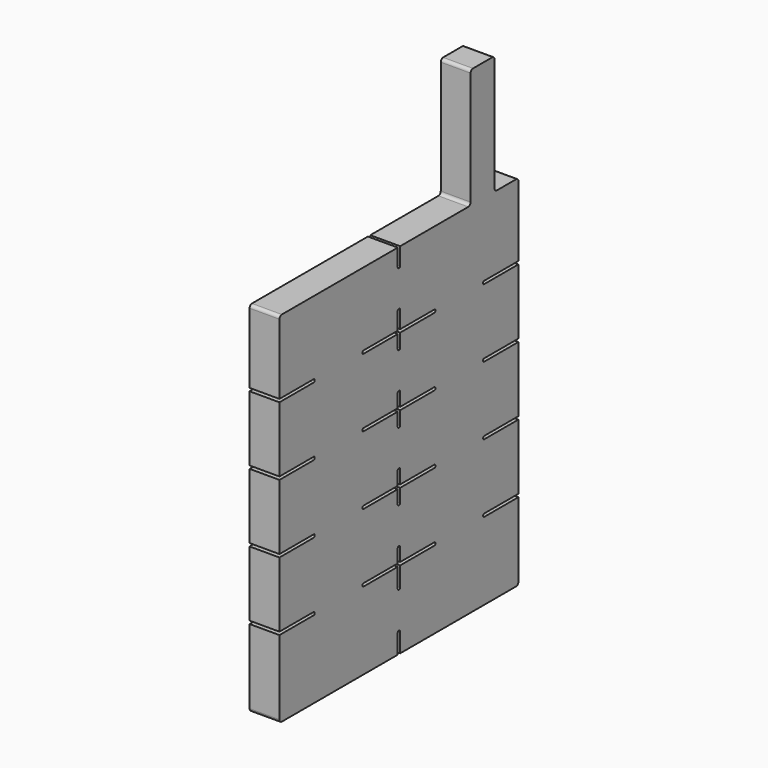
from build123d import *

# Parameters (mm, degrees)
F1_DEPTH = 5
F2_R     = 0.5
F3_R     = 0.5
F4_R     = 0.5
F5_R     = 0.2


# Not quite as in the source:
# - a feature names something its author has since deleted; it is built from what else it names


with BuildPart() as f1:
    # F0 (on Right) → F1 (new body)
    with BuildSketch(Plane.YZ):
        Polygon((11.5, 0), (0, 0), (0, -12.238), (7.3750000447, -12.238), (7.3750000447, -12.738), (0, -12.738), (0, -23.672), (7.3750000447, -23.672), (7.3750000447, -24.172), (0, -24.172), (0, -35.106), (7.3750000447, -35.106), (7.3750000447, -35.606), (0, -35.606), (0, -46.54), (7.3750000447, -46.54), (7.3750000447, -47.04), (0, -47.04), (0, -60), (24.75, -60), (24.75, -56.52), (25.25, -56.52), (25.25, -60), (50, -60), (50, -47.04), (42.6249988377, -47.04), (42.6249988377, -46.54), (50, -46.54), (50, -35.606), (42.6249988377, -35.606), (42.6249988377, -35.106), (50, -35.106), (50, -24.172), (42.6249988377, -24.172), (42.6249988377, -23.672), (50, -23.672), (50, -12.738), (42.6249988377, -12.738), (42.6249988377, -12.238), (50, -12.238), (50, 0), (45, 0), (45, 15), (45, 19.999999553), (40, 19.999999553), (40, 15), (40, 0), (37.625, 0), (35.125, 0), (25.25, 0), (25.25, -1.304), (25.25, -3.119), (24.75, -3.119), (24.75, 0), (14.875, 0), (12.375, 0), align=None)
        Polygon((25.25, -44.073), (25.25, -46.54), (32.625, -46.54), (32.625, -47.04), (25.25, -47.04), (25.25, -50.52), (24.75, -50.52), (24.75, -47.04), (17.375, -47.04), (17.375, -46.54), (24.75, -46.54), (24.75, -44.073), align=None, mode=Mode.SUBTRACT)
        Polygon((25.25, -32.639), (25.25, -35.106), (32.625, -35.106), (32.625, -35.606), (25.25, -35.606), (25.25, -38.073), (24.75, -38.073), (24.75, -35.606), (17.375, -35.606), (17.375, -35.106), (24.75, -35.106), (24.75, -32.639), align=None, mode=Mode.SUBTRACT)
        Polygon((25.25, -21.205), (25.25, -23.672), (32.625, -23.672), (32.625, -24.172), (25.25, -24.172), (25.25, -26.639), (24.75, -26.639), (24.75, -24.172), (17.375, -24.172), (17.375, -23.672), (24.75, -23.672), (24.75, -21.205), align=None, mode=Mode.SUBTRACT)
        Polygon((25.25, -9.119), (25.25, -12.238), (32.625, -12.238), (32.625, -12.738), (25.25, -12.738), (25.25, -15.205), (24.75, -15.205), (24.75, -12.738), (17.375, -12.738), (17.375, -12.238), (24.75, -12.238), (24.75, -9.119), align=None, mode=Mode.SUBTRACT)
    extrude(amount=F1_DEPTH)

    # F2
    f2_edges = [f1.edges().sort_by_distance(p)[0] for p in [
        (2.5, 0, 0),
        (2.5, 50, 0),
        (2.5, 50, -60),
        (2.5, 0, -60),
    ]]
    fillet(f2_edges, radius=F2_R)

    # F3
    f3_edges = [f1.edges().sort_by_distance(p)[0] for p in [
        (2.5, 45, 20),
        (2.5, 40, 20),
    ]]
    fillet(f3_edges, radius=F3_R)

    # F4
    f4_edges = [f1.edges().sort_by_distance(p)[0] for p in [
        (2.5, 40, 0),
        (2.5, 45, 0),
    ]]
    fillet(f4_edges, radius=F4_R)

    # F5
    f5_edges = [f1.edges().sort_by_distance(p)[0] for p in [
        (2.5, 25.25, -3.119),
        (2.5, 24.75, -3.119),
        (2.5, 42.624999, -12.238),
        (2.5, 42.624999, -12.738),
        (2.5, 42.624999, -23.672),
        (2.5, 42.624999, -24.172),
        (2.5, 42.624999, -35.106),
        (2.5, 42.624999, -35.606),
        (2.5, 42.624999, -46.54),
        (2.5, 42.624999, -47.04),
        (2.5, 24.75, -56.52),
        (2.5, 25.25, -56.52),
        (2.5, 24.75, -50.52),
        (2.5, 25.25, -50.52),
        (2.5, 32.625, -47.04),
        (2.5, 32.625, -46.54),
        (2.5, 25.25, -44.073),
        (2.5, 24.75, -44.073),
        (2.5, 17.375, -46.54),
        (2.5, 17.375, -47.04),
        (2.5, 24.75, -38.073),
        (2.5, 25.25, -38.073),
        (2.5, 32.625, -35.606),
        (2.5, 32.625, -35.106),
        (2.5, 25.25, -32.639),
        (2.5, 24.75, -32.639),
        (2.5, 17.375, -35.606),
        (2.5, 17.375, -35.106),
        (2.5, 17.375, -23.672),
        (2.5, 17.375, -24.172),
        (2.5, 24.75, -26.639),
        (2.5, 25.25, -26.639),
        (2.5, 32.625, -24.172),
        (2.5, 32.625, -23.672),
        (2.5, 25.25, -21.205),
        (2.5, 24.75, -21.205),
        (2.5, 17.375, -12.238),
        (2.5, 17.375, -12.738),
        (2.5, 24.75, -15.205),
        (2.5, 25.25, -15.205),
        (2.5, 32.625, -12.738),
        (2.5, 32.625, -12.238),
        (2.5, 25.25, -9.119),
        (2.5, 24.75, -9.119),
        (2.5, 7.375, -12.738),
        (2.5, 7.375, -24.172),
        (2.5, 7.375, -12.238),
        (2.5, 7.375, -23.672),
        (2.5, 7.375, -46.54),
        (2.5, 7.375, -35.106),
        (2.5, 7.375, -35.606),
        (2.5, 7.375, -47.04),
    ]]
    fillet(f5_edges, radius=F5_R)


solid = f1.part
